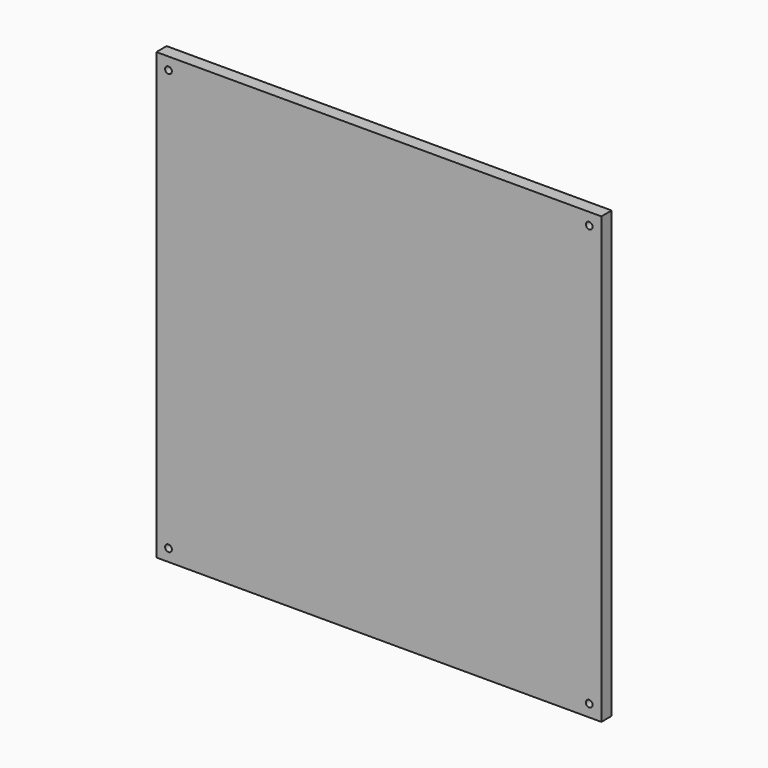
from build123d import *

# Parameters (mm, degrees)
F0_W            = 330.2
F0_H            = 330.2
F1_DEPTH        = 9.525
F3_D            = 5
F3_COPIES_COUNT = 4


# Not quite as in the source:
# - a pattern or mirror of a feature is missing from the dataset's text; its kind, count and spacing are read off the source's solid


with BuildPart() as f1:
    # F0 (on Front) → F1 (new body)
    with BuildSketch(Plane.XZ):
        with Locations((165.1, 165.1)):
            Rectangle(F0_W, F0_H)
    extrude(amount=F1_DEPTH)

    # F3 (through all)
    with Locations(Plane(origin=(0, 0, 0), x_dir=(-1, 0, 0), z_dir=(0, 1, 0))):
        with Locations((-321.2197438789, 8.9802561211)):
            f3 = Hole(F3_D / 2)

    # F3_copies: F3 ×4 about axis
    f3_copies_axis = Axis((165.1, 0, 165.1), (0, 1, 0))
    for i in range(1, F3_COPIES_COUNT):
        add(f3.rotate(f3_copies_axis, i * 360 / F3_COPIES_COUNT), mode=Mode.SUBTRACT)


solid = f1.part
